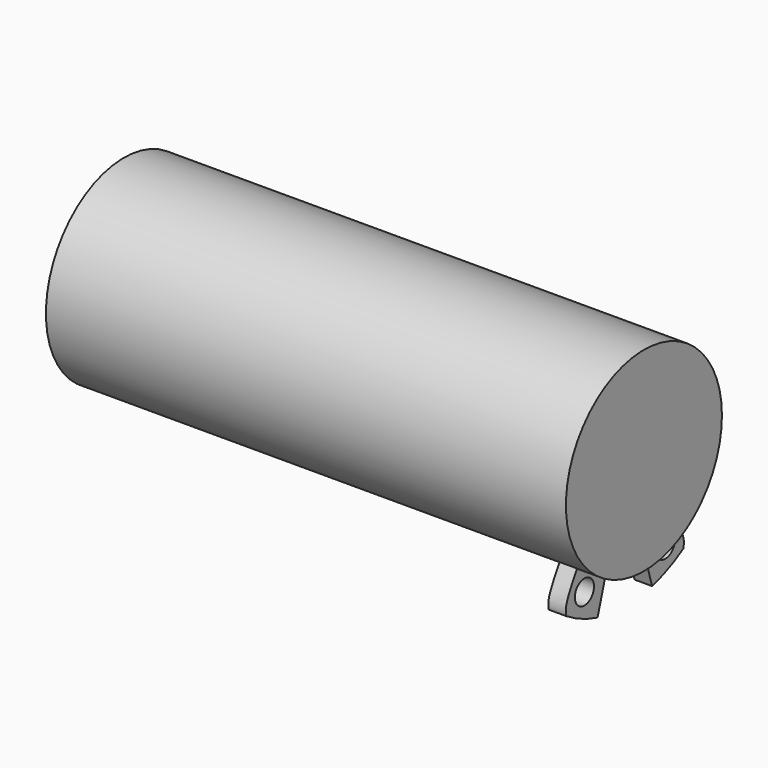
from build123d import *

# Parameters (mm, degrees)
F0_R     = 4.7625
F1_DEPTH = 12.7
F2_W     = 0.8572917432
F2_H     = 3.6824136041
F5_R     = 0.5850055068
F6_DEPTH = 25.4


with BuildPart() as f1:
    # F0 (on Right) → F1 (new body)
    with BuildSketch(Plane.YZ):
        Circle(F0_R)
    extrude(amount=F1_DEPTH)

    # F4: F1 across plane


with BuildPart() as f3:
    # F2 (on Top) → F3 (revolve)
    with BuildSketch(Plane.XY):
        with Locations((11.3397957757, 4.7545640264)):
            Rectangle(F2_W, F2_H)
    revolve(axis=Axis((11.6089691874, 0, 0), (-1, 0, 0)))

    # F5 (on face) → F6 (cut)
    with BuildSketch(Plane.YZ.offset(11.7684416473)):
        with BuildLine():
            ThreePointArc((0.6035996611, -2.850143464), (0, -2.9133572243), (-0.6035996611, -2.850143464))
            Line((-0.6035996611, -2.850143464), (-1.6657512694, -6.3819640809))
            ThreePointArc((-1.6657512694, -6.3819640809), (0, -6.5957708284), (1.6657512694, -6.3819640809))
            Line((1.6657512694, -6.3819640809), (0.6035996611, -2.850143464))
        make_face()
        with BuildLine():
            ThreePointArc((6.5957708284, 0), (-3.156008436, 5.7917012676), (-3.5755357392, -5.5425388586))
            add(Edge.make_bspline(
                [(-3.5755357392, -5.5425388586), (-3.6011746585, -5.4133196937), (-3.6721900788, -5.0271716823), (-3.1553549859, -4.1579107621), (-2.8186723188, -3.5900480977)],
                knots=[0, 0, 0, 0, 0.3399807639, 1, 1, 1, 1], degree=3))
            ThreePointArc((-2.8186723188, -3.5900480977), (0, 4.5643574558), (2.8186723188, -3.5900480977))
            add(Edge.make_bspline(
                [(3.5755357392, -5.5425388586), (3.6011746585, -5.4133196937), (3.6721900788, -5.0271716823), (3.1553549859, -4.1579107621), (2.8186723188, -3.5900480977)],
                knots=[0, 0, 0, 0, 0.3399807639, 1, 1, 1, 1], degree=3))
            ThreePointArc((3.5755357392, -5.5425388586), (5.7917012676, -3.156008436), (6.5957708284, 0))
        make_face()
        with Locations((-2.4692576844, -4.9510691315)):
            Circle(F5_R)
        with Locations((2.4692576844, -4.9510691315)):
            Circle(F5_R)
    extrude(amount=-F6_DEPTH, mode=Mode.SUBTRACT)


with BuildPart() as f1_1:
    add(f1.part)
    add(f1.part.mirror(Plane.YZ))


solid = Compound([f3.part, f1_1.part])
